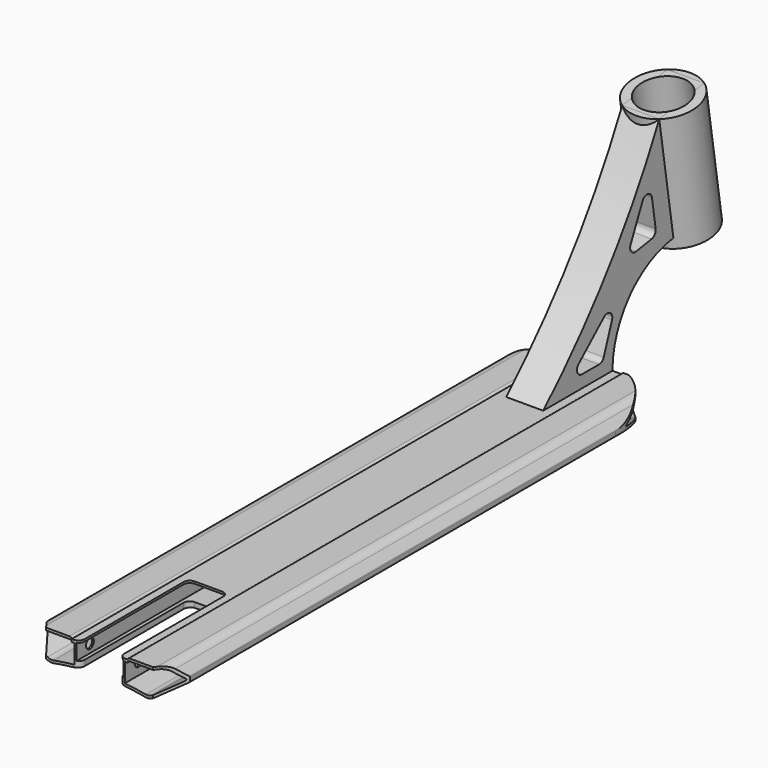
from build123d import *

# Parameters (mm, degrees)
F1_DEPTH       = 250
F2_W           = 38
F2_H           = 13
F3_DEPTH       = 250
F4_T1_DEPTH    = 509.3674969976
F5_R           = 9
F6_R           = 1
F8_DEPTH       = 500.001
F10_DEPTH      = 22.2193051812
F10_DEPTH_BACK = 1.301
F12_DEPTH      = 22.219305294
F12_DEPTH_BACK = 1.3010001
F13_T1_DEPTH   = 1.7268039449
F13_T6_DEPTH   = 17.0390927402
F13_S7_R       = 200
F13_T8_DEPTH   = 11
F13_T12_DEPTH  = 17.0390927402
F13_S13_R      = 200
F13_T14_DEPTH  = 11
F13_T15_DEPTH  = 26.731632452
F15_DEPTH      = 15
F16_R          = 27.5
F17_DEPTH      = 100
F19_D          = 40
F21_D          = 8
F21_DEPTH      = 50
F21_TIP        = 2.4034424761
F23_DEPTH      = 42.5010001
F23_DEPTH_BACK = 72.5010001
F24_T1_DEPTH   = 30
F24_T3_DEPTH   = 29.5366784866


# Not quite as in the source:
# - a fillet or chamfer that OpenCascade refuses, or shapes differently, is made with other operations: its cross-section is extruded or revolved along the edge and cut away or added


with BuildPart() as f1:
    # F0 (on Front) → F1 (new body, symmetric)
    with BuildSketch(Plane.XZ):
        with BuildLine():
            Line((22.5, 0), (0, 0))
            Line((0, 0), (-22.5, 0))
            Line((-22.5, 0), (-22.5, 1.3))
            Line((-22.5, 1.3), (-49.1090036882, 1.3))
            Line((-49.1090036882, 1.3), (-57.5, -8.7))
            Line((-57.5, -8.7), (-57.5, -12.7))
            Line((-57.5, -12.7), (-40.1794919243, -22.7))
            ThreePointArc((-40.1794919243, -22.7), (0, -18.6224551416), (40.1794919243, -22.7))
            Line((40.1794919243, -22.7), (57.5, -12.7))
            Line((57.5, -12.7), (57.5, -8.7))
            Line((57.5, -8.7), (49.1090036882, 1.3))
            Line((49.1090036882, 1.3), (22.5, 1.3))
            Line((22.5, 1.3), (22.5, 0))
        make_face()
    extrude(amount=F1_DEPTH, both=True)

    # F2 (on Front) → F3 (cut, symmetric)
    with BuildSketch(Plane.XZ):
        with Locations((0, -8.2268039449)):
            Rectangle(F2_W, F2_H)
    extrude(amount=F3_DEPTH, both=True, mode=Mode.SUBTRACT)

    # F4: fillet of radius 2 on 2 edges, made by hand

    # F4_s2 → F4_t1 (cut)
    with BuildSketch(Plane.XZ.offset(-254.6837484988)):
        with BuildLine():
            ThreePointArc((24.3734993995, 1.3), (23.2333239744, 0.9431676725), (22.5, 0))
            Line((22.5, 0), (22.5, 1.3))
            Line((22.5, 1.3), (24.3734993995, 1.3))
        make_face()
        with BuildLine():
            ThreePointArc((-24.3734993995, 1.3), (-23.2333239744, 0.9431676725), (-22.5, 0))
            Line((-22.5, 0), (-22.5, 1.3))
            Line((-22.5, 1.3), (-24.3734993995, 1.3))
        make_face()
    extrude(amount=F4_T1_DEPTH, mode=Mode.SUBTRACT)

    # F5
    f5_edges = [f1.edges().sort_by_distance(p)[0] for p in [
        (-49.109004, 0, 1.3),
        (49.109004, 0, 1.3),
        (40.179492, 0, -22.7),
        (-40.179492, 0, -22.7),
    ]]
    fillet(f5_edges, radius=F5_R)

    # F6
    f6_edges = [f1.edges().sort_by_distance(p)[0] for p in [
        (-57.5, 0, -8.7),
        (-57.5, 0, -12.7),
        (57.5, 0, -8.7),
        (57.5, 0, -12.7),
    ]]
    fillet(f6_edges, radius=F6_R)

    # F7 (on face) → F8 (cut, through all)
    with BuildSketch(Plane.XZ.offset(250)):
        with BuildLine():
            ThreePointArc((-37.3093701274, -20.0978700124), (-28.8874083403, -18.698675567), (-20.4138456833, -17.6566000706))
            Line((-20.4138456833, -17.6566000706), (-20.4138456833, -2.3003034743))
            Line((-20.4138456833, -2.3003034743), (-22.4138456833, -2.3003034743))
            ThreePointArc((-22.4138456833, -2.3003034743), (-23.1084683824, -1.1509046105), (-24.3734993995, -0.7))
            Line((-24.3734993995, -0.7), (-44.9122347648, -0.7))
            ThreePointArc((-44.9122347648, -0.7), (-47.870562597, -1.3558454907), (-50.2745458667, -3.2004867322))
            Line((-50.2745458667, -3.2004867322), (-55.9308095341, -9.9413592785))
            ThreePointArc((-55.9308095341, -9.9413592785), (-56.149572844, -10.7577950659), (-55.664765091, -11.450172292))
            Line((-55.664765091, -11.450172292), (-42.1022690923, -19.2804830077))
            ThreePointArc((-42.1022690923, -19.2804830077), (-39.7790673433, -20.1186780608), (-37.3093701274, -20.0978700124))
        make_face()
        with BuildLine():
            Line((22.4138456833, -2.3003034743), (20.4138456833, -2.3003034743))
            Line((20.4138456833, -2.3003034743), (20.4138456833, -17.6566000706))
            ThreePointArc((20.4138456833, -17.6566000706), (28.8874083403, -18.698675567), (37.3093701274, -20.0978700124))
            ThreePointArc((37.3093701274, -20.0978700124), (39.7790673433, -20.1186780608), (42.1022690923, -19.2804830077))
            Line((42.1022690923, -19.2804830077), (55.664765091, -11.450172292))
            ThreePointArc((55.664765091, -11.450172292), (56.149572844, -10.7577950659), (55.9308095341, -9.9413592785))
            Line((55.9308095341, -9.9413592785), (50.2745458667, -3.2004867322))
            ThreePointArc((50.2745458667, -3.2004867322), (47.870562597, -1.3558454907), (44.9122347648, -0.7))
            Line((44.9122347648, -0.7), (24.3734993995, -0.7))
            ThreePointArc((24.3734993995, -0.7), (23.1084683824, -1.1509046105), (22.4138456833, -2.3003034743))
        make_face()
    extrude(amount=-F8_DEPTH, mode=Mode.SUBTRACT)

    # F9 (on Top) → F10 (cut, two sides)
    with BuildSketch(Plane.XY) as f10_sk:
        with BuildLine():
            ThreePointArc((-57.5, 200), (0, 257.5), (57.5, 200))
            Line((57.5, 200), (57.5, 280))
            Line((57.5, 280), (-57.5, 280))
            Line((-57.5, 280), (-57.5, 200))
        make_face()
    extrude(amount=-F10_DEPTH, mode=Mode.SUBTRACT)
    extrude(f10_sk.sketch, amount=F10_DEPTH_BACK, mode=Mode.SUBTRACT)

    # F11 (on Top) → F12 (cut, two sides)
    with BuildSketch(Plane.XY) as f12_sk:
        Polygon((16, -140), (-16, -140), (-16, -250), (-43.2975540478, -250), (-68, -216), (-68, -346), (68, -346), (68, -216), (43.2975540478, -250), (16, -250), align=None)
    extrude(amount=-F12_DEPTH, mode=Mode.SUBTRACT)
    extrude(f12_sk.sketch, amount=F12_DEPTH_BACK, mode=Mode.SUBTRACT)

    # F13: fillet of radius 5 on 6 edges, made by hand

    # F13_s2 → F13_t1 (join)
    with BuildSketch(Plane.XY.offset(-1.7268039449)):
        with BuildLine():
            ThreePointArc((-10.9990343146, -139.9996), (-14.5355339059, -141.4644660941), (-16.0004, -145.0009656854))
            Line((-16.0004, -145.0009656854), (-16.5005365685, -145.0009656854))
            ThreePointArc((-16.5005365685, -145.0009656854), (-16.5001365685, -142.5004828427), (-16.5001365685, -140))
            Line((-16.5001365685, -140), (-16, -139.4998634315))
            ThreePointArc((-16, -139.4998634315), (-13.4995171573, -139.4998634315), (-10.9990343146, -139.4994634315))
            Line((-10.9990343146, -139.4994634315), (-10.9990343146, -139.9996))
        make_face()
        with BuildLine():
            ThreePointArc((16.0004, -145.0009656854), (14.5355339059, -141.4644660941), (10.9990343146, -139.9996))
            Line((10.9990343146, -139.9996), (10.9990343146, -139.4994634315))
            ThreePointArc((10.9990343146, -139.4994634315), (13.4995171573, -139.4998634315), (16, -139.4998634315))
            Line((16, -139.4998634315), (16.5001365685, -140))
            ThreePointArc((16.5001365685, -140), (16.5001365685, -142.5004828427), (16.5005365685, -145.0009656854))
            Line((16.5005365685, -145.0009656854), (16.0004, -145.0009656854))
        make_face()
    extrude(amount=F13_T1_DEPTH)


with BuildPart() as f13_tool4:
    # F13_s5 → F13_t6 (new body)
    with BuildSketch(Plane.XY.offset(-31.7658966851)):
        with BuildLine():
            ThreePointArc((-16.0004, -145.0009656854), (-14.5355339059, -141.4644660941), (-10.9990343146, -139.9996))
            Line((-10.9990343146, -139.9996), (-10.9990343146, -139.4994634315))
            ThreePointArc((-10.9990343146, -139.4994634315), (-13.4995171573, -139.4998634315), (-16, -139.4998634315))
            Line((-16, -139.4998634315), (-16.5001365685, -140))
            ThreePointArc((-16.5001365685, -140), (-16.5001365685, -142.5004828427), (-16.5005365685, -145.0009656854))
            Line((-16.5005365685, -145.0009656854), (-16.0004, -145.0009656854))
        make_face()
    extrude(amount=F13_T6_DEPTH)

    # F13_s7 → F13_t8 (cut, symmetric)
    with BuildSketch(Plane.XZ.offset(142.3)):
        with Locations((0, -218.6224551416)):
            Circle(F13_S7_R)
    extrude(amount=F13_T8_DEPTH, both=True, mode=Mode.SUBTRACT)


with BuildPart() as f1_1:
    add(f1.part)

    # F13_t3: union F13_tool4
    add(f13_tool4.part)


with BuildPart() as f13_tool10:
    # F13_s11 → F13_t12 (new body)
    with BuildSketch(Plane.XY.offset(-14.7268039449)):
        with BuildLine():
            ThreePointArc((16.0004, -145.0009656854), (14.5355339059, -141.4644660941), (10.9990343146, -139.9996))
            Line((10.9990343146, -139.9996), (10.9990343146, -139.4994634315))
            ThreePointArc((10.9990343146, -139.4994634315), (13.4995171573, -139.4998634315), (16, -139.4998634315))
            Line((16, -139.4998634315), (16.5001365685, -140))
            ThreePointArc((16.5001365685, -140), (16.5001365685, -142.5004828427), (16.5005365685, -145.0009656854))
            Line((16.5005365685, -145.0009656854), (16.0004, -145.0009656854))
        make_face()
    extrude(amount=-F13_T12_DEPTH)

    # F13_s13 → F13_t14 (cut, symmetric)
    with BuildSketch(Plane.XZ.offset(142.3)):
        with Locations((0, -218.6224551416)):
            Circle(F13_S13_R)
    extrude(amount=F13_T14_DEPTH, both=True, mode=Mode.SUBTRACT)


with BuildPart() as f1_2:
    add(f1_1.part)

    # F13_t9: union F13_tool10
    add(f13_tool10.part)

    # F13_s16 → F13_t15 (cut)
    with BuildSketch(Plane.XY.offset(-14.2292181985)):
        with BuildLine():
            ThreePointArc((-21.0009656854, -250.0004), (-17.4644660941, -248.5355339059), (-15.9996, -244.9990343146))
            Line((-15.9996, -244.9990343146), (-15.4994634315, -244.9990343146))
            ThreePointArc((-15.4994634315, -244.9990343146), (-15.4998634315, -247.4995171573), (-15.4998634315, -250))
            Line((-15.4998634315, -250), (-16, -250.5001365685))
            ThreePointArc((-16, -250.5001365685), (-18.5004828427, -250.5001365685), (-21.0009656854, -250.5005365685))
            Line((-21.0009656854, -250.5005365685), (-21.0009656854, -250.0004))
        make_face()
        with BuildLine():
            ThreePointArc((21.0009656854, -250.0004), (17.4644660941, -248.5355339059), (15.9996, -244.9990343146))
            Line((15.9996, -244.9990343146), (15.4994634315, -244.9990343146))
            ThreePointArc((15.4994634315, -244.9990343146), (15.4998634315, -247.4995171573), (15.4998634315, -250))
            Line((15.4998634315, -250), (16, -250.5001365685))
            ThreePointArc((16, -250.5001365685), (18.5004828427, -250.5001365685), (21.0009656854, -250.5005365685))
            Line((21.0009656854, -250.5005365685), (21.0009656854, -250.0004))
        make_face()
    extrude(amount=F13_T15_DEPTH, mode=Mode.SUBTRACT)

    # F14 (on Right) → F15 (join, symmetric)
    with BuildSketch(Plane.YZ):
        with BuildLine():
            Line((180, 0), (250, 0))
            ThreePointArc((250, 0), (267.6550746197, 46.4758946867), (311.7145367693, 69.5079211245))
            Line((311.7145367693, 69.5079211245), (313.0254460068, 61.2311659405))
            Line((313.0254460068, 61.2311659405), (358.4591096742, 68.4271513323))
            Line((358.4591096742, 68.4271513323), (342.8156631702, 167.1959853919))
            Line((342.8156631702, 167.1959853919), (297.3819995028, 160))
            ThreePointArc((297.3819995028, 160), (245.9666940414, 74.662277853), (180, 0))
        make_face()
    extrude(amount=F15_DEPTH, both=True)

    # F16 (on face) → F17 (join, through all)
    with BuildSketch(Plane(origin=(0, -17.4439040266, 110.1364754698), x_dir=(1, 0, 0), z_dir=(0, -0.156434465, 0.9876883406))):
        with Locations((0, 341.7502480182)):
            Circle(F16_R)
    extrude(amount=-F17_DEPTH)

    # F19 (through all)
    with Locations(Plane(origin=(0, -17.4439040266, 110.1364754698), x_dir=(1, 0, 0), z_dir=(0, -0.156434465, 0.9876883406))):
        with Locations((0, 341.7502480182)):
            Hole(F19_D / 2)

    # F21 (one way)
    with BuildSketch(Plane.YZ.offset(20.4138456833)):
        with Locations((-236, -7.7170047426)):
            Circle(F21_D / 2)
    extrude(amount=-F21_DEPTH, mode=Mode.SUBTRACT)
    with Locations(Plane.YZ.offset(20.4138456833)):
        with Locations((-236, -7.7170047426)):
            with Locations((0, 0, -(F21_DEPTH + F21_TIP / 2))):  # 118° drill point
                Cone(0, F21_D / 2, F21_TIP, mode=Mode.SUBTRACT)

    # F22 (on face) → F23 (cut, two sides)
    with BuildSketch(Plane.YZ.offset(15)) as f23_sk:
        Polygon((240, 10), (256.378660542, 55), (206, 10), align=None)
        Polygon((287.3447062809, 123.5418922598), (264.4720060955, 73.7903590501), (294.4720060955, 78.5418922598), align=None)
    extrude(amount=F23_DEPTH, mode=Mode.SUBTRACT)
    extrude(f23_sk.sketch, amount=-F23_DEPTH_BACK, mode=Mode.SUBTRACT)

    # F24: fillet of radius 5 on 8 edges, made by hand

    # F24_s2 → F24_t1 (join)
    with BuildSketch(Plane.YZ.offset(-15)):
        with BuildLine():
            ThreePointArc((289.5335643925, 77.7597199346), (292.7964770392, 79.7592353761), (293.6898337703, 83.4803339628))
            Line((293.6898337703, 83.4803339628), (294.4720060955, 78.5418922598))
            Line((294.4720060955, 78.5418922598), (289.5335643925, 77.7597199346))
        make_face()
        with BuildLine():
            ThreePointArc((236.498962309, 10), (239.3668444907, 10.9042397786), (241.1974254129, 13.2898992834))
            Line((241.1974254129, 13.2898992834), (240, 10))
            Line((240, 10), (236.498962309, 10))
        make_face()
        with BuildLine():
            ThreePointArc((241.5480825238, 41.752803595), (247.683139761, 42.1634412906), (249.5774091206, 36.3137152957))
            Line((249.5774091206, 36.3137152957), (256.378660542, 55))
            Line((256.378660542, 55), (241.5480825238, 41.752803595))
        make_face()
        with BuildLine():
            ThreePointArc((289.9280459811, 107.2313273149), (285.6720755071, 111.4023593082), (280.4467012633, 108.5377028579))
            Line((280.4467012633, 108.5377028579), (287.3447062809, 123.5418922598))
            Line((287.3447062809, 123.5418922598), (289.9280459811, 107.2313273149))
        make_face()
        with BuildLine():
            ThreePointArc((215.7723267178, 18.7289875827), (214.4317376575, 13.2174369455), (219.1031902107, 10))
            Line((219.1031902107, 10), (206, 10))
            Line((206, 10), (215.7723267178, 18.7289875827))
        make_face()
        with BuildLine():
            ThreePointArc((273.6995688245, 75.2518614085), (268.932372103, 77.1704387831), (268.3744934845, 82.2788509797))
            Line((268.3744934845, 82.2788509797), (264.4720060955, 73.7903590501))
            Line((264.4720060955, 73.7903590501), (273.6995688245, 75.2518614085))
        make_face()
    extrude(amount=F24_T1_DEPTH)

    # F24_s4 → F24_t3 (cut)
    with BuildSketch(Plane.XY.offset(-31.7634824315)):
        with BuildLine():
            ThreePointArc((21, -250), (17.4644660941, -248.5355339059), (16, -245))
            Line((16, -245), (16, -250))
            Line((16, -250), (21, -250))
        make_face()
        with BuildLine():
            ThreePointArc((-21, -250), (-17.4644660941, -248.5355339059), (-16, -245))
            Line((-16, -245), (-16, -250))
            Line((-16, -250), (-21, -250))
        make_face()
    extrude(amount=F24_T3_DEPTH, mode=Mode.SUBTRACT)


solid = f1_2.part
